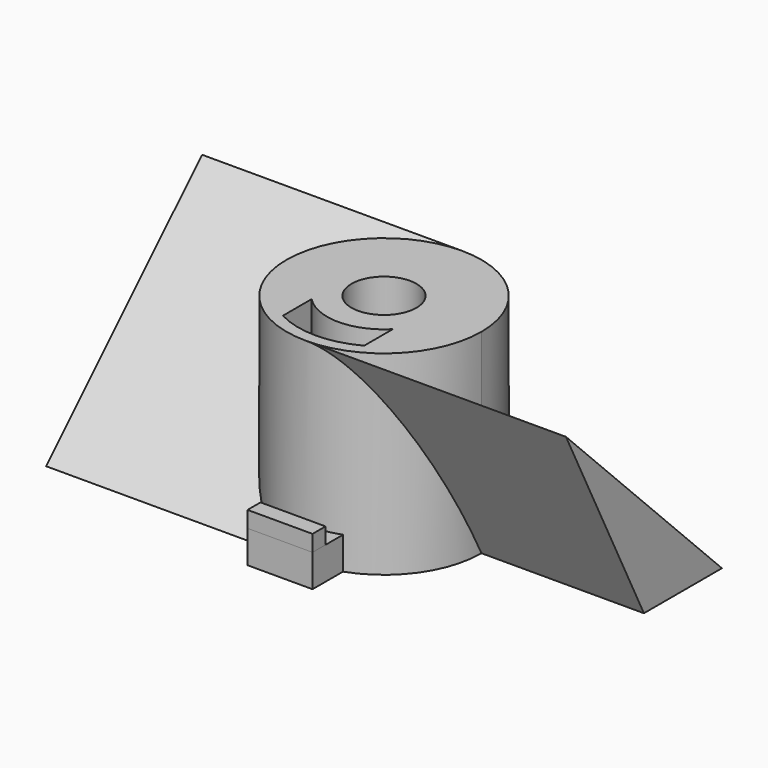
from build123d import *
from build123d import SkipClean  # not in build123d's __all__

# Parameters (mm, degrees)
F0_R      = 7.62
F1_DEPTH  = 15.24
F3_DEPTH  = 20.32
F5_COUNT  = 2
F6_W      = 5.0799995622
F6_H      = 2.54
F7_DEPTH  = 10.16
F8_W      = 5.0799995622
F8_H      = 1.27
F9_DEPTH  = 1.27
F10_R     = 2.54
F11_DEPTH = 13.97
F13_DEPTH = 25.4


with BuildPart() as f1:
    # F0 (on Top) → F1 (new body)
    with BuildSketch(Plane.XY):
        Circle(F0_R)
    extrude(amount=F1_DEPTH)



with BuildPart() as f3:
    # F2 (on Right) → F3 (new body)
    with BuildSketch(Plane.YZ):
        Polygon((-7.62, 15.24), (0, 0), (7.62, 0), align=None)
    extrude(amount=F3_DEPTH)


with BuildPart() as f1_1:
    add(f1.part, clean=False)

    with SkipClean():  # cleaning this boolean's faces spoils the solid; the shape is the same uncleaned
        add(f3.part)  # F5 merges F3
    # F5: F3 ×2 about axis
    f5_axis = Axis((0, 0, 17.5851359963), (0, 0, 1))
    with SkipClean():  # cleaning this boolean's faces spoils the solid; the shape is the same uncleaned
        for i in range(1, F5_COUNT):
            add(f3.part.rotate(f5_axis, i * 360 / F5_COUNT), clean=False)

    # F6 (on Front) → F7 (join)
    with BuildSketch(Plane.XZ):
        with Locations((0, 1.27)):
            Rectangle(F6_W, F6_H)
    with SkipClean():  # cleaning this boolean's faces spoils the solid; the shape is the same uncleaned
        extrude(amount=F7_DEPTH)

    # F8 (on face) → F9 (join)
    with BuildSketch(Plane.XY.offset(2.54)):
        with Locations((0, -9.525)):
            Rectangle(F8_W, F8_H)
    with SkipClean():  # cleaning this boolean's faces spoils the solid; the shape is the same uncleaned
        extrude(amount=F9_DEPTH)

    # F10 (on face) → F11 (cut)
    with BuildSketch(Plane.XY.offset(15.24)):
        Circle(F10_R)
    with SkipClean():  # cleaning this boolean's faces spoils the solid; the shape is the same uncleaned
        extrude(amount=-F11_DEPTH, mode=Mode.SUBTRACT)

    # F12 (on face) → F13 (cut)
    with BuildSketch(Plane.XY.offset(15.24)):
        with BuildLine():
            ThreePointArc((3.175, -3.1108519733), (0, -4.445), (-3.175, -3.1108519733))
            Line((-3.175, -3.1108519733), (-3.175, -5.9048519733))
            ThreePointArc((-3.175, -5.9048519733), (0, -6.7043196394), (3.175, -5.9048519733))
            Line((3.175, -5.9048519733), (3.175, -3.1108519733))
        make_face()
    with SkipClean():  # cleaning this boolean's faces spoils the solid; the shape is the same uncleaned
        extrude(amount=-F13_DEPTH, mode=Mode.SUBTRACT)


solid = f1_1.part
